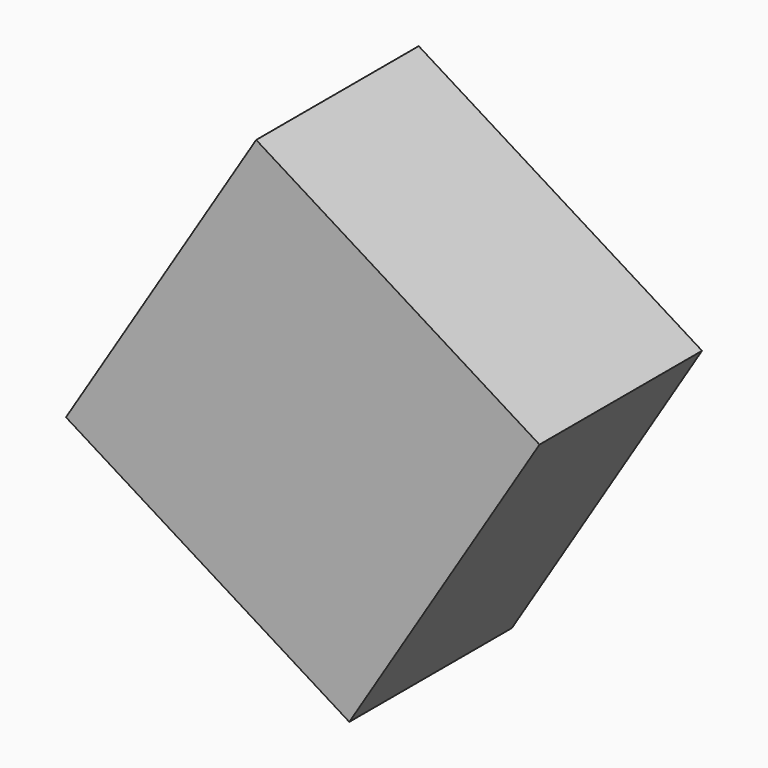
from build123d import *

# Parameters (mm, degrees)
F1_E2_W  = 76.8327403991
F1_E2_H  = 46.7958282679
F2_DEPTH = 82.9861517996


with BuildPart() as f2:
    # F1_E2 (on explicit) → F2 (new body)
    with BuildSketch(Plane(origin=(41.1237664521, 0, 0), x_dir=(-0.8493090083, 0, 0.5278960204), z_dir=(0.5278960204, 0, 0.8493090083))):
        with Locations((38.4163701995, 23.397914134)):
            Rectangle(F1_E2_W, F1_E2_H)
    extrude(amount=F2_DEPTH)


solid = f2.part
